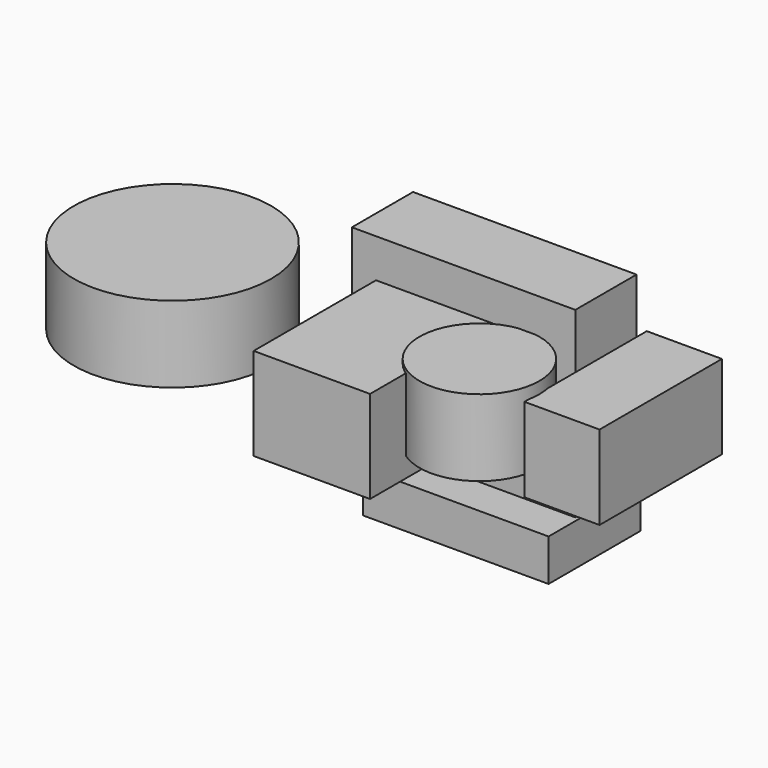
from build123d import *

# Parameters (mm, degrees)
F0_W      = 77.3211158812
F0_H      = 61.4438680932
F1_DEPTH  = 50.8
F2_W      = 49.9155819416
F2_H      = 55.8106014505
F3_DEPTH  = 101.6
F4_W      = 123.2228167355
F4_H      = 27.7765095234
F5_DEPTH  = 76.2
F6_W      = 148.441709578
F6_H      = 149.5107635856
F7_DEPTH  = 50.8
F8_DEPTH  = 101.6
F9_R      = 65.5812572733
F10_DEPTH = 50.8
F11_DEPTH = 50.8
F14_R     = 39.8220041085
F15_DEPTH = 50.8


# Not quite as in the source:
# - the program builds the solid bodies; features that only make, move or delete a surface that nothing else refers to are left out


with BuildPart() as f1:
    # F0 (on Front) → F1 (new body)
    with BuildSketch(Plane.XZ):
        with Locations((-17.1259511262, 17.4385928549)):
            Rectangle(F0_W, F0_H)
    extrude(amount=F1_DEPTH)


with BuildPart() as f3:
    # F2 (on Front) → F3 (new body)
    with BuildSketch(Plane.XZ):
        with Locations((108.3693355322, 15.127654653)):
            Rectangle(F2_W, F2_H)
    extrude(amount=F3_DEPTH)


with BuildPart() as f5:
    # F4 (on Front) → F5 (new body)
    with BuildSketch(Plane.XZ):
        with Locations((17.5292175263, -61.3352879882)):
            Rectangle(F4_W, F4_H)
    extrude(amount=F5_DEPTH)


with BuildPart() as f7:
    # F6 (on Front) → F7 (new body)
    with BuildSketch(Plane.XZ):
        with Locations((2.3990385234, -0.8346028626)):
            Rectangle(F6_W, F6_H)
    extrude(amount=F7_DEPTH)


with BuildPart() as f8:
    # F8 (new): a face of the model
    f8_faces = [f1.part.faces().sort_by_distance(p)[0] for p in [
        (-17.1259511262, -50.8, 17.4385928549),
    ]]
    extrude(f8_faces, amount=F8_DEPTH)


with BuildPart() as f10:
    # F9 (on Top) → F10 (new body)
    with BuildSketch(Plane.XY):
        with Locations((-161.6249978542, -87.4381959438)):
            Circle(F9_R)
    extrude(amount=F10_DEPTH)


with BuildPart() as f11:
    # F0 (on Front) → F11 (new body)
    with BuildSketch(Plane.XZ):
        with Locations((-17.1259511262, 17.4385928549)):
            Rectangle(F0_W, F0_H)
    extrude(amount=F11_DEPTH)


with BuildPart() as f15:
    # F14 (on Top) → F15 (new body)
    with BuildSketch(Plane.XY):
        with Locations((44.3835146725, -90.1619270444)):
            Circle(F14_R)
    extrude(amount=F15_DEPTH)


solid = Compound([f1.part, f3.part, f5.part, f7.part, f8.part, f10.part, f11.part, f15.part])
